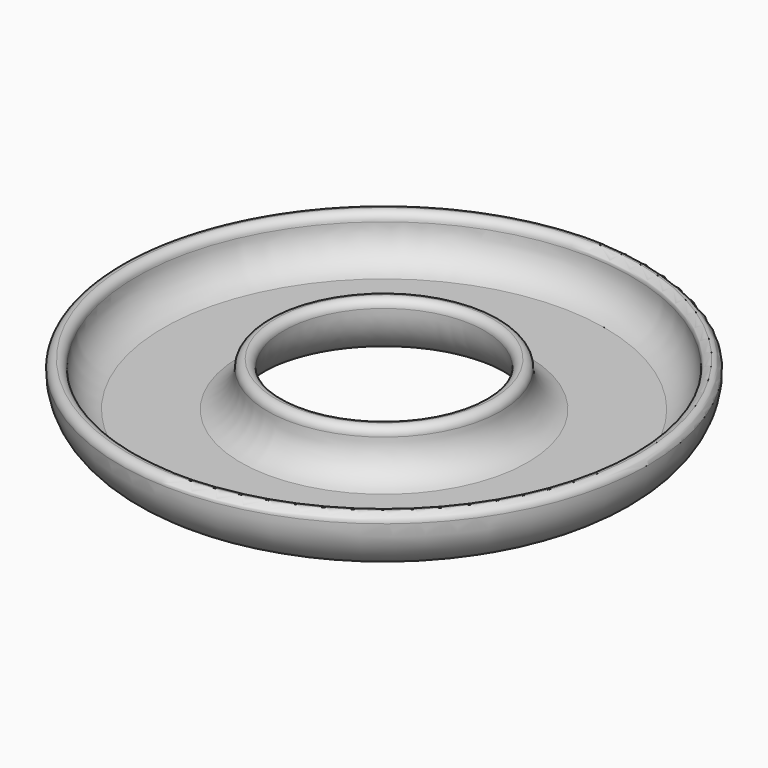
from build123d import *


# Not quite as in the source:
# - a fillet or chamfer that OpenCascade refuses, or shapes differently, is made with other operations: its cross-section is extruded or revolved along the edge and cut away or added


with BuildPart() as f1:
    # F0 (on Front) → F1 (revolve)
    with BuildSketch(Plane.XZ):
        with BuildLine():
            ThreePointArc((5, 3), (5.3955149615, 1.0970099744), (7, 0))
            Line((7, 0), (11, 0))
            ThreePointArc((11, 0), (12.6044850385, 1.0970099744), (13, 3))
            Line((13, 3), (12.1811805528, 3))
            ThreePointArc((12.1811805528, 3), (11.9981299392, 1.6359991878), (10.9049185685, 0.8))
            Line((10.9049185685, 0.8), (7.0950814315, 0.8))
            ThreePointArc((7.0950814315, 0.8), (6.0018700608, 1.6359991878), (5.8188194472, 3))
            Line((5.8188194472, 3), (5, 3))
        make_face()
    revolve(axis=Axis((0, 0, -1.7576739192), (0, 0, -1)))

    # F2: fillet of radius 0.4 on 4 edges, made by hand

    # F2_s1 → F2_t2 (revolve, cut)
    with BuildSketch(Plane.XZ):
        with BuildLine():
            ThreePointArc((12.6403148098, 3), (12.3535922949, 2.8789089447), (12.2404674395, 2.5889509972))
            Line((12.2404674395, 2.5889509972), (12.2324704921, 2.5887300171))
            ThreePointArc((12.2324704921, 2.5887300171), (12.21480048, 2.7950490393), (12.1734471026, 2.9979521355))
            Line((12.1734471026, 2.9979521355), (12.1811805528, 3.008))
            Line((12.1811805528, 3.008), (12.6403148098, 3.008))
            Line((12.6403148098, 3.008), (12.6403148098, 3))
        make_face()
    revolve(axis=Axis((0, 0, 3), (0, 0, -1)), mode=Mode.SUBTRACT)

    # F2_s3 → F2_t4 (revolve, cut)
    with BuildSketch(Plane.XZ):
        with BuildLine():
            ThreePointArc((5.7595325605, 2.5889509972), (5.6464077051, 2.8789089447), (5.3596851902, 3))
            Line((5.3596851902, 3), (5.3596851902, 3.008))
            Line((5.3596851902, 3.008), (5.8188194472, 3.008))
            Line((5.8188194472, 3.008), (5.8265528974, 2.9979521355))
            ThreePointArc((5.8265528974, 2.9979521355), (5.78519952, 2.7950490393), (5.7675295079, 2.5887300171))
            Line((5.7675295079, 2.5887300171), (5.7595325605, 2.5889509972))
        make_face()
    revolve(axis=Axis((0, 0, 3), (0, 0, -1)), mode=Mode.SUBTRACT)

    # F2_s5 → F2_t6 (revolve, cut)
    with BuildSketch(Plane.XZ):
        with BuildLine():
            ThreePointArc((5.3596851902, 3), (5.0807762454, 2.8867225149), (4.9598378199, 2.6110490028))
            Line((4.9598378199, 2.6110490028), (4.9518408724, 2.6112699829))
            ThreePointArc((4.9518408724, 2.6112699829), (4.9646389685, 2.8071022728), (4.9921266285, 3.0014177524))
            Line((4.9921266285, 3.0014177524), (5, 3.008))
            Line((5, 3.008), (5.3596851902, 3.008))
            Line((5.3596851902, 3.008), (5.3596851902, 3))
        make_face()
    revolve(axis=Axis((0, 0, 3), (0, 0, -1)), mode=Mode.SUBTRACT)

    # F2_s7 → F2_t8 (revolve, cut)
    with BuildSketch(Plane.XZ):
        with BuildLine():
            ThreePointArc((13.0401621801, 2.6110490028), (12.9192237546, 2.8867225149), (12.6403148098, 3))
            Line((12.6403148098, 3), (12.6403148098, 3.008))
            Line((12.6403148098, 3.008), (13, 3.008))
            Line((13, 3.008), (13.0078733715, 3.0014177524))
            ThreePointArc((13.0078733715, 3.0014177524), (13.0353610315, 2.8071022728), (13.0481591276, 2.6112699829))
            Line((13.0481591276, 2.6112699829), (13.0401621801, 2.6110490028))
        make_face()
    revolve(axis=Axis((0, 0, 3), (0, 0, -1)), mode=Mode.SUBTRACT)


solid = f1.part
